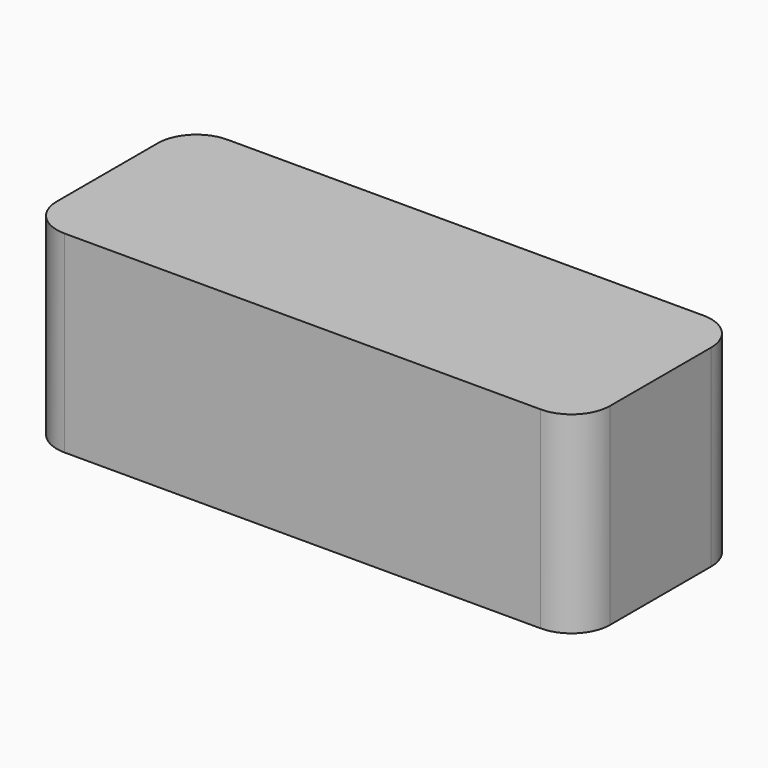
from build123d import *

# Parameters (mm, degrees)
F1_W     = 71.7420950532
F1_H     = 26.3687837869
F2_DEPTH = 25
F3_R     = 5


# Not quite as in the source:
# - a feature of the source that left no trace in its solid (it failed there, or was rolled back) is left out


with BuildPart() as f2:
    # F1 (on Top) → F2 (new body)
    with BuildSketch(Plane.XY):
        with Locations((-0.274553895, -31.835465692)):
            Rectangle(F1_W, F1_H)
    extrude(amount=F2_DEPTH)

    # F3
    f3_edges = [f2.edges().sort_by_distance(p)[0] for p in [
        (-36.145601, -45.019858, 12.5),
        (35.596494, -45.019858, 12.5),
        (35.596494, -18.651074, 12.5),
        (-36.145601, -18.651074, 12.5),
    ]]
    fillet(f3_edges, radius=F3_R)


solid = f2.part
